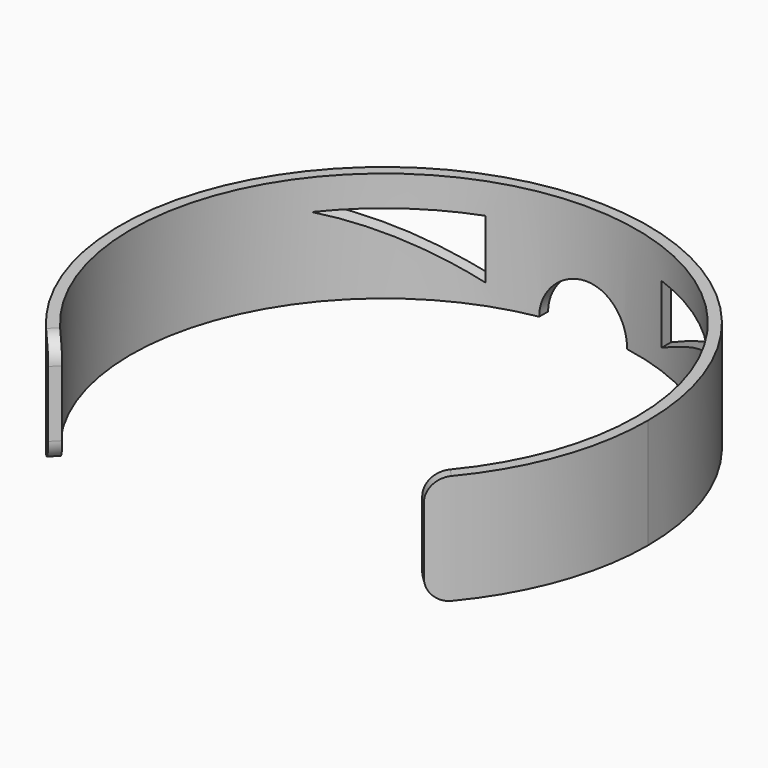
from build123d import *

# Parameters (mm, degrees)
F0_R     = 60
F0_R_2   = 57.5
F1_DEPTH = 25
F2_R     = 10
F3_DEPTH = 60.001
F5_DEPTH = 60.0010001012
F7_DEPTH = 25.0010001
F8_R     = 5


# Not quite as in the source:
# - a feature names something its author has since deleted; it is built from what else it names


with BuildPart() as f1:
    # F0 (on Top) → F1 (new body)
    with BuildSketch(Plane.XY):
        Circle(F0_R)
        Circle(F0_R_2, mode=Mode.SUBTRACT)
    extrude(amount=F1_DEPTH)

    # F2 (on Front) → F3 (cut, through all)
    with BuildSketch(Plane.XZ):
        Circle(F2_R)
    extrude(amount=-F3_DEPTH, mode=Mode.SUBTRACT)

    # F4 (on Front) → F5 (cut, through all)
    with BuildSketch(Plane.XZ):
        Polygon((-20, 4.6551390551), (-20, 18.0386640131), (-45.0213760883, 18.0386640131), align=None)
        Polygon((45.0213760883, 18.0386640131), (20, 18.0386640131), (20, 4.6551390551), align=None)
    extrude(amount=-F5_DEPTH, mode=Mode.SUBTRACT)

    # F6 (on Top) → F7 (cut, through all)
    with BuildSketch(Plane.XY):
        Polygon((66.0135835631, -64.9920968146), (0, 0), (-63.9864164369, -64.9920968146), align=None)
    extrude(amount=F7_DEPTH, mode=Mode.SUBTRACT)

    # F8
    f8_edges = [f1.edges().sort_by_distance(p)[0] for p in [
        (-41.217352, -41.865169, 25),
        (-41.217352, -41.865169, 0),
        (41.865169, -41.217352, 25),
        (41.865169, -41.217352, 0),
    ]]
    fillet(f8_edges, radius=F8_R)


solid = f1.part
